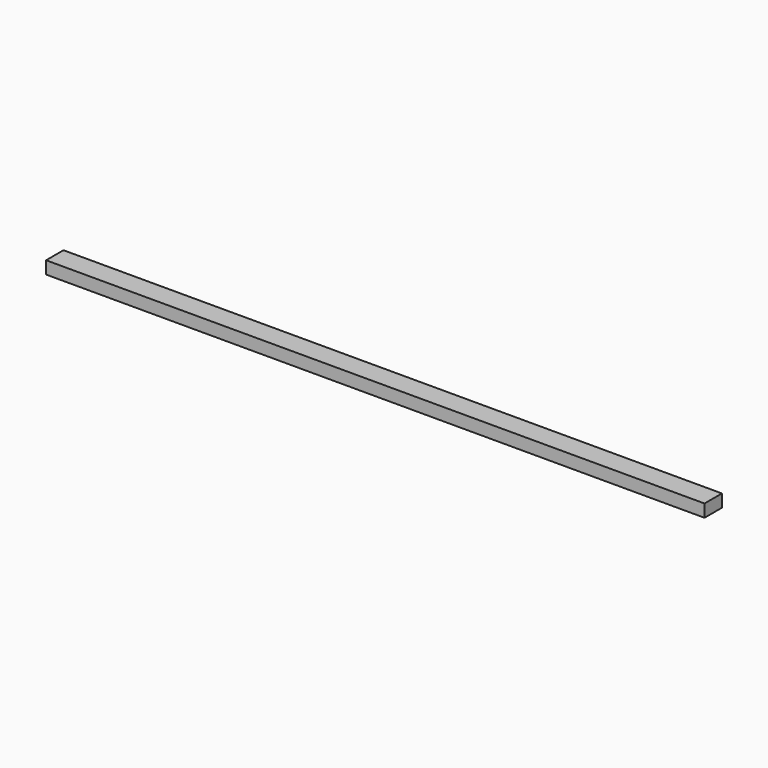
from build123d import *

# Parameters (mm, degrees)
F1_W     = 251.5227198601
F1_H     = 13.4035423398
F2_DEPTH = 88.9
F3_DEPTH = 38.1
F4_DEPTH = 2438.4


# Not quite as in the source:
# - a feature of the source that left no trace in its solid (it failed there, or was rolled back) is left out


with BuildPart() as f2:
    # F1 (on face) → F2 (new body)
    with BuildSketch(Plane.XZ):
        with Locations((54.7012239695, 18.0854015052)):
            Rectangle(F1_W, F1_H)
    extrude(amount=F2_DEPTH)

    # F3 (add): a face of the model
    f3_faces = [f2.faces().sort_by_distance(p)[0] for p in [
        (54.7012239695, -44.45, 24.7871726751),
    ]]
    extrude(f3_faces, amount=F3_DEPTH)

    # F4 (add): a face of the model
    f4_faces = [f2.faces().sort_by_distance(p)[0] for p in [
        (180.4625838995, -44.45, 37.1354015052),
    ]]
    extrude(f4_faces, amount=F4_DEPTH)


solid = f2.part
